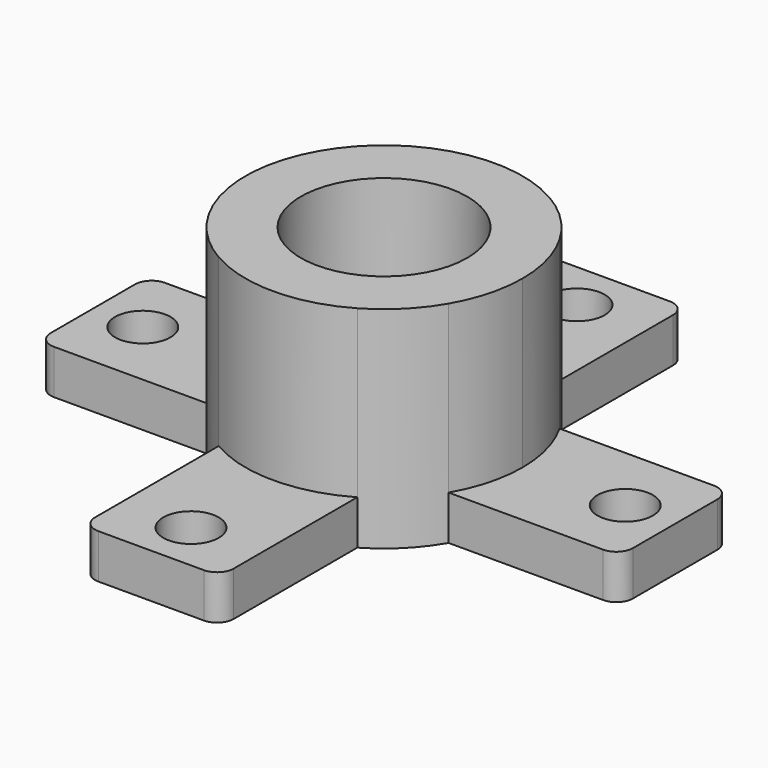
from build123d import *

# Parameters (mm, degrees)
F0_R     = 1
F0_W     = 5
F0_H     = 5
F1_DEPTH = 1.6
F2_R     = 3
F3_DEPTH = 6
F4_DEPTH = 1.6
F5_R     = 2.5
F6_DEPTH = 1.6


with BuildPart() as f1:
    # F0 (on Top) → F1 (new body)
    with BuildSketch(Plane.XY):
        with BuildLine():
            ThreePointArc((10.5, 1.9), (10.3242640687, 2.3242640687), (9.9, 2.5))
            Line((9.9, 2.5), (2.5, 2.5))
            Line((2.5, 2.5), (2.5, -2.5))
            Line((2.5, -2.5), (9.9, -2.5))
            ThreePointArc((9.9, -2.5), (10.3242640687, -2.3242640687), (10.5, -1.9))
            Line((10.5, -1.9), (10.5, 1.9))
        make_face()
        with Locations((8.7, 0)):
            Circle(F0_R, mode=Mode.SUBTRACT)
        Rectangle(F0_W, F0_H)
        with BuildLine():
            Line((-2.5, 2.5), (2.5, 2.5))
            Line((2.5, 2.5), (2.5, 9.9))
            ThreePointArc((2.5, 9.9), (2.3242640687, 10.3242640687), (1.9, 10.5))
            Line((1.9, 10.5), (-1.9, 10.5))
            ThreePointArc((-1.9, 10.5), (-2.3242640687, 10.3242640687), (-2.5, 9.9))
            Line((-2.5, 9.9), (-2.5, 2.5))
        make_face()
        with Locations((0, 8.7)):
            Circle(F0_R, mode=Mode.SUBTRACT)
        with BuildLine():
            Line((-2.5, -2.5), (-2.5, 2.5))
            Line((-2.5, 2.5), (-9.9, 2.5))
            ThreePointArc((-9.9, 2.5), (-10.3242640687, 2.3242640687), (-10.5, 1.9))
            Line((-10.5, 1.9), (-10.5, -1.9))
            ThreePointArc((-10.5, -1.9), (-10.3242640687, -2.3242640687), (-9.9, -2.5))
            Line((-9.9, -2.5), (-2.5, -2.5))
        make_face()
        with Locations((-8.7, 0)):
            Circle(F0_R, mode=Mode.SUBTRACT)
        with BuildLine():
            Line((2.5, -9.9), (2.5, -2.5))
            Line((2.5, -2.5), (-2.5, -2.5))
            Line((-2.5, -2.5), (-2.5, -9.9))
            ThreePointArc((-2.5, -9.9), (-2.3242640687, -10.3242640687), (-1.9, -10.5))
            Line((-1.9, -10.5), (1.9, -10.5))
            ThreePointArc((1.9, -10.5), (2.3242640687, -10.3242640687), (2.5, -9.9))
        make_face()
        with Locations((0, -8.7)):
            Circle(F0_R, mode=Mode.SUBTRACT)
    extrude(amount=F1_DEPTH)

    # F2 (on face) → F3 (join)
    with BuildSketch(Plane.XY.offset(1.6)):
        with BuildLine():
            ThreePointArc((4.3301270189, -2.5), (4.8296291314, -1.2940952255), (5, 0))
            ThreePointArc((5, 0), (4.8296291314, 1.2940952255), (4.3301270189, 2.5))
            Line((4.3301270189, 2.5), (2.5, 2.5))
            Line((2.5, 2.5), (2.5, 4.3301270189))
            ThreePointArc((2.5, 4.3301270189), (0, 5), (-2.5, 4.3301270189))
            Line((-2.5, 4.3301270189), (-2.5, 2.5))
            Line((-2.5, 2.5), (-4.3301270189, 2.5))
            ThreePointArc((-4.3301270189, 2.5), (-5, 0), (-4.3301270189, -2.5))
            Line((-4.3301270189, -2.5), (-2.5, -2.5))
            Line((-2.5, -2.5), (-2.5, -4.3301270189))
            ThreePointArc((-2.5, -4.3301270189), (0, -5), (2.5, -4.3301270189))
            Line((2.5, -4.3301270189), (2.5, -2.5))
            Line((2.5, -2.5), (4.3301270189, -2.5))
        make_face()
        Circle(F2_R, mode=Mode.SUBTRACT)
        with BuildLine():
            ThreePointArc((-4.3301270189, -2.5), (-3.5355339059, -3.5355339059), (-2.5, -4.3301270189))
            Line((-2.5, -4.3301270189), (-2.5, -2.5))
            Line((-2.5, -2.5), (-4.3301270189, -2.5))
        make_face()
        with BuildLine():
            ThreePointArc((2.5, -4.3301270189), (3.5355339059, -3.5355339059), (4.3301270189, -2.5))
            Line((4.3301270189, -2.5), (2.5, -2.5))
            Line((2.5, -2.5), (2.5, -4.3301270189))
        make_face()
        with BuildLine():
            Line((2.5, 2.5), (4.3301270189, 2.5))
            ThreePointArc((4.3301270189, 2.5), (3.5355339059, 3.5355339059), (2.5, 4.3301270189))
            Line((2.5, 4.3301270189), (2.5, 2.5))
        make_face()
        with BuildLine():
            Line((-2.5, 2.5), (-2.5, 4.3301270189))
            ThreePointArc((-2.5, 4.3301270189), (-3.5355339059, 3.5355339059), (-4.3301270189, 2.5))
            Line((-4.3301270189, 2.5), (-2.5, 2.5))
        make_face()
    extrude(amount=F3_DEPTH)

    # F4 (add, through all): faces of the model
    f4_faces = [f1.faces().sort_by_distance(p)[0] for p in [
        (-3.1629509292, 3.1629509292, 1.6),
        (3.1629509292, 3.1629509292, 1.6),
        (-3.1629509292, -3.1629509292, 1.6),
        (3.1629509292, -3.1629509292, 1.6),
    ]]
    extrude(f4_faces, amount=F4_DEPTH)

    # F5 (on face) → F6 (cut, through all)
    with BuildSketch(Plane.XY.offset(1.6)):
        Circle(F5_R)
    extrude(amount=-F6_DEPTH, mode=Mode.SUBTRACT)


solid = f1.part
